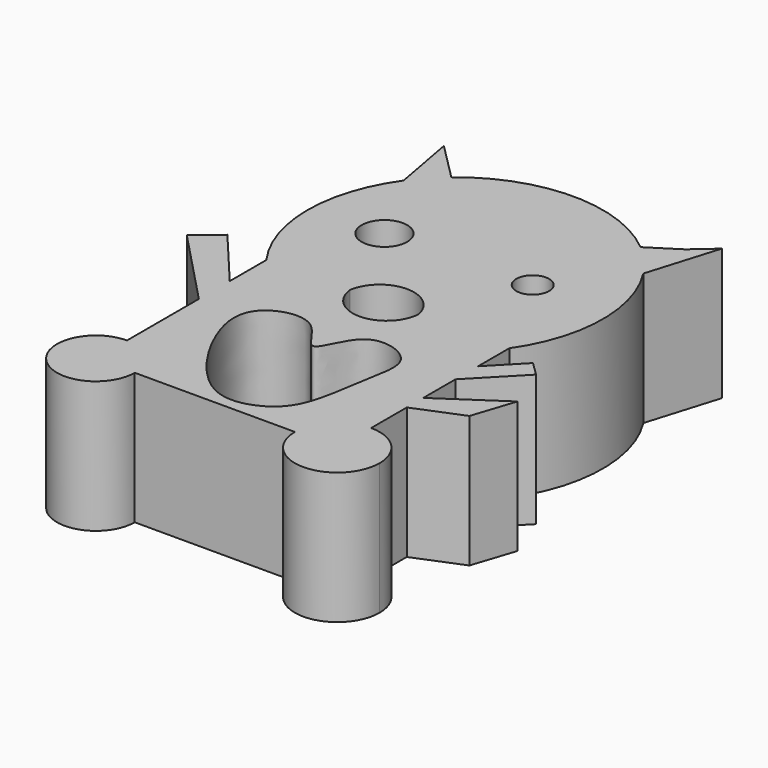
from build123d import *

# Parameters (mm, degrees)
F0_R     = 4.7418950376
F0_R_2   = 3.4234930155
F1_DEPTH = 27.432


# Not quite as in the source:
# - a feature names something its author has since deleted; it is built from what else it names


with BuildPart() as f1:
    # F0 (on Top) → F1 (new body)
    with BuildSketch(Plane.XY):
        with BuildLine():
            Line((25.2953674644, 5.6984800103), (25.2953674644, 13.8353250349))
            ThreePointArc((25.2953674644, 13.8353250349), (30.7668689842, 30.8370384198), (25.8731804788, 48.0139822607))
            Line((25.8731804788, 48.0139822607), (30.3728617728, 62.8549531102))
            Line((30.3728617728, 62.8549531102), (25.8731804788, 58.917734772))
            Line((25.8731804788, 58.917734772), (19.7135022724, 54.9844578476))
            ThreePointArc((19.7135022724, 54.9844578476), (0, 62.1284381568), (-19.7135022724, 54.9844578476))
            Line((-19.7135022724, 54.9844578476), (-27.5605618954, 62.8549531102))
            Line((-27.5605618954, 62.8549531102), (-25.0568710899, 49.2184152222))
            ThreePointArc((-25.0568710899, 49.2184152222), (-30.7712265115, 31.3083269796), (-25.0000394881, 13.4164707571))
            Line((-25.0000394881, 13.4164707571), (-25.0000394881, 10.5883115903))
            Line((-25.0000394881, 10.5883115903), (-25.0000394881, 3.8822568022))
            Line((-25.0000394881, 3.8822568022), (-35.5061925948, 16.4002254605))
            Line((-35.5061925948, 16.4002254605), (-40.5666477737, 12.1530573815))
            Line((-40.5666477737, 12.1530573815), (-25.0000394881, -4.1650086641))
            Line((-25.0000394881, -4.1650086641), (-25.0000394881, -22.8893524268))
            ThreePointArc((-25.0000394881, -22.8893524268), (-19.2725639904, -25.2617504561), (-16.9001659611, -30.9892259538))
            Line((-16.9001659611, -30.9892259538), (16.4749322786, -30.9892259538))
            ThreePointArc((16.4749322786, -30.9892259538), (19.0583779315, -24.7522364209), (25.2953674644, -22.168790768))
            Line((25.2953674644, -22.168790768), (25.2953674644, -12.8828799352))
            Line((25.2953674644, -12.8828799352), (35.1309105754, -8.8592460379))
            Line((35.1309105754, -8.8592460379), (38.0368679762, 0))
            Line((38.0368679762, 0), (25.2953674644, -8.5769504594))
            Line((25.2953674644, -8.5769504594), (25.2953674644, -0.1902780768))
            Line((25.2953674644, -0.1902780768), (34.4973343106, 9.2992545014))
            Line((34.4973343106, 9.2992545014), (31.5543487668, 12.1530573815))
            Line((31.5543487668, 12.1530573815), (25.2953674644, 5.6984800103))
        make_face()
        with BuildLine():
            add(Edge.make_bspline(
                [(0, -5.4839896038), (-1.2402732611, -5.6900448164), (-4.274773093, 2.3105176673), (-14.1907812378, 0.9256060054), (-19.0134260803, -7.4792396235), (-5.4071900703, -30.3441353211), (6.5664135103, -28.1751540776), (12.3781283881, -22.4582417314), (13.6895995956, -9.0366780223), (16.3381064135, 0.8586419268), (3.4670177632, 4.8861409136), (1.3437918836, -5.2607361233), (0, -5.4839896038)],
                knots=[0, 0, 0, 0, 0.0862123206, 0.176335532, 0.2645289981, 0.4179663282, 0.5169948409, 0.6026118794, 0.7186193313, 0.8125731341, 0.9065920226, 1, 1, 1, 1], degree=3))
        make_face(mode=Mode.SUBTRACT)
        with Locations((-15.8350989223, 32.7182896435)):
            Circle(F0_R, mode=Mode.SUBTRACT)
        with BuildLine():
            ThreePointArc((6.2948795967, 13.9413382858), (-0.643780333, 7.3596103039), (-7.7878357843, 13.7178031728))
            ThreePointArc((-7.7878357843, 13.7178031728), (-0.8402846529, 19.7393853242), (6.2948795967, 13.9413382858))
        make_face(mode=Mode.SUBTRACT)
        with Locations((14.3421432003, 33.6124300957)):
            Circle(F0_R_2, mode=Mode.SUBTRACT)
        with BuildLine():
            ThreePointArc((34.1158026503, -30.9892259538), (31.5323569973, -24.7522364209), (25.2953674644, -22.168790768))
            Line((25.2953674644, -22.168790768), (25.2953674644, -30.9892259538))
            Line((25.2953674644, -30.9892259538), (16.4749322786, -30.9892259538))
            ThreePointArc((16.4749322786, -30.9892259538), (25.2953674644, -39.8096611397), (34.1158026503, -30.9892259538))
        make_face()
        with BuildLine():
            Line((25.2953674644, -30.9892259538), (25.2953674644, -22.168790768))
            ThreePointArc((25.2953674644, -22.168790768), (19.0583779315, -24.7522364209), (16.4749322786, -30.9892259538))
            Line((16.4749322786, -30.9892259538), (25.2953674644, -30.9892259538))
        make_face()
        with BuildLine():
            ThreePointArc((-25.0000394881, -22.8893524268), (-30.7275149858, -36.7167014515), (-16.9001659611, -30.9892259538))
            ThreePointArc((-16.9001659611, -30.9892259538), (-19.2725639904, -25.2617504561), (-25.0000394881, -22.8893524268))
        make_face()
    extrude(amount=F1_DEPTH)


solid = f1.part
